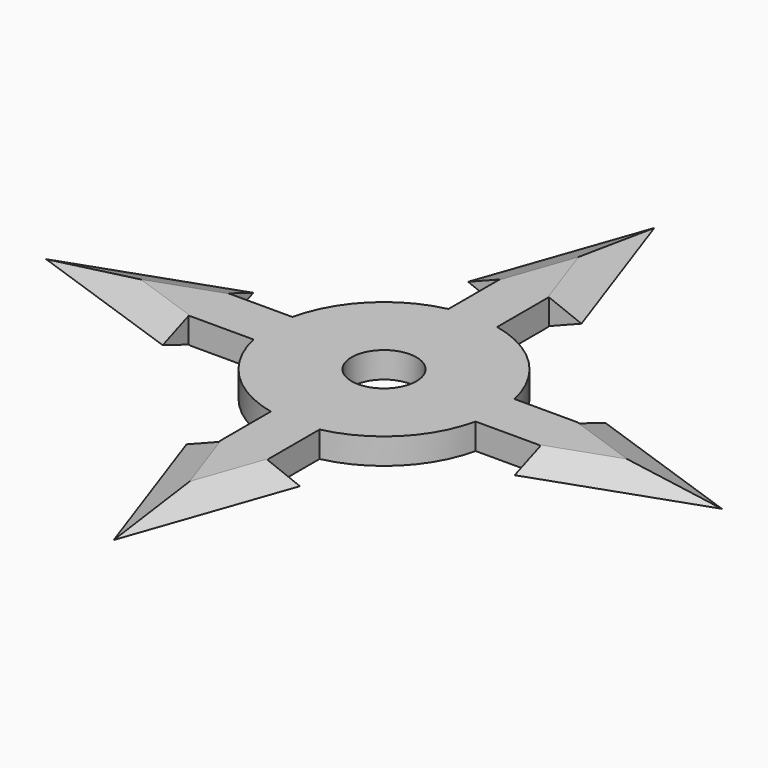
from build123d import *

# Parameters (mm, degrees)
F0_R         = 5
F1_DEPTH     = 2
F2_SIZE      = 1.99999
F3_T1_DEPTH  = 34.8509927222
F3_T3_DEPTH  = 34.8509927222
F3_T5_DEPTH  = 34.8509927222
F3_T7_DEPTH  = 34.8509927222
F3_T9_DEPTH  = 34.8509927222
F3_T11_DEPTH = 34.8509927222
F3_T13_DEPTH = 34.8509927222
F3_T15_DEPTH = 34.8509927222


# Not quite as in the source:
# - a fillet or chamfer that OpenCascade refuses, or shapes differently, is made with other operations: its cross-section is extruded or revolved along the edge and cut away or added
# - a fillet or chamfer is up to 0.001 mm smaller than in the source, because OpenCascade refuses the exact size


with BuildPart() as f1:
    # F0 (on Top) → F1 (new body, symmetric)
    with BuildSketch(Plane.XY):
        with BuildLine():
            ThreePointArc((17.093492914, -3.75), (17.3980764166, -1.8859843591), (17.5, 0))
            ThreePointArc((17.5, 0), (17.3980764166, 1.8859843591), (17.093492914, 3.75))
            ThreePointArc((17.093492914, 3.75), (12.3743686708, 12.3743686708), (3.75, 17.093492914))
            ThreePointArc((3.75, 17.093492914), (0, 17.5), (-3.75, 17.093492914))
            ThreePointArc((-3.75, 17.093492914), (-12.3743686708, 12.3743686708), (-17.093492914, 3.75))
            ThreePointArc((-17.093492914, 3.75), (-17.5, 0), (-17.093492914, -3.75))
            ThreePointArc((-17.093492914, -3.75), (-12.3743686708, -12.3743686708), (-3.75, -17.093492914))
            ThreePointArc((-3.75, -17.093492914), (0, -17.5), (3.75, -17.093492914))
            ThreePointArc((3.75, -17.093492914), (12.3743686708, -12.3743686708), (17.093492914, -3.75))
        make_face()
        Circle(F0_R, mode=Mode.SUBTRACT)
        with BuildLine():
            ThreePointArc((-17.093492914, -3.75), (-17.5, 0), (-17.093492914, 3.75))
            Line((-17.093492914, 3.75), (-27.093492914, 3.75))
            Line((-27.093492914, 3.75), (-27.093492914, -3.75))
            Line((-27.093492914, -3.75), (-17.093492914, -3.75))
        make_face()
        Polygon((-27.093492914, -3.75), (-27.093492914, 3.75), (-27.093492914, 8.75), (-52.093492914, 0), (-27.093492914, -8.75), align=None)
        with BuildLine():
            ThreePointArc((-3.75, 17.093492914), (0, 17.5), (3.75, 17.093492914))
            Line((3.75, 17.093492914), (3.75, 27.093492914))
            Line((3.75, 27.093492914), (-3.75, 27.093492914))
            Line((-3.75, 27.093492914), (-3.75, 17.093492914))
        make_face()
        Polygon((-3.75, 27.093492914), (3.75, 27.093492914), (8.75, 27.093492914), (0, 52.093492914), (-8.75, 27.093492914), align=None)
        Polygon((27.093492914, 8.75), (27.093492914, 3.75), (27.093492914, -3.75), (27.093492914, -8.75), (52.093492914, 0), align=None)
        Polygon((8.75, -27.093492914), (3.75, -27.093492914), (-3.75, -27.093492914), (-8.75, -27.093492914), (0, -52.093492914), align=None)
        with BuildLine():
            Line((3.75, -27.093492914), (3.75, -17.093492914))
            ThreePointArc((3.75, -17.093492914), (0, -17.5), (-3.75, -17.093492914))
            Line((-3.75, -17.093492914), (-3.75, -27.093492914))
            Line((-3.75, -27.093492914), (3.75, -27.093492914))
        make_face()
        with BuildLine():
            ThreePointArc((17.093492914, 3.75), (17.3980764166, 1.8859843591), (17.5, 0))
            ThreePointArc((17.5, 0), (17.3980764166, -1.8859843591), (17.093492914, -3.75))
            Line((17.093492914, -3.75), (27.093492914, -3.75))
            Line((27.093492914, -3.75), (27.093492914, 3.75))
            Line((27.093492914, 3.75), (17.093492914, 3.75))
        make_face()
    extrude(amount=F1_DEPTH, both=True)

    # F2 (size 2 in the source; OpenCascade refuses exactly that, so slightly less here)
    f2_edges = [f1.edges().sort_by_distance(p)[0] for p in [
        (4.375, -39.593493, 2),
        (-4.375, -39.593493, 2),
        (4.375, -39.593493, -2),
        (-4.375, -39.593493, -2),
        (39.593493, -4.375, -2),
        (39.593493, -4.375, 2),
        (39.593493, 4.375, 2),
        (-39.593493, -4.375, 2),
        (-39.593493, -4.375, -2),
        (-4.375, 39.593493, 2),
        (4.375, 39.593493, 2),
        (39.593493, 4.375, -2),
        (4.375, 39.593493, -2),
        (-39.593493, 4.375, 2),
        (-39.593493, 4.375, -2),
        (-4.375, 39.593493, -2),
    ]]
    chamfer(f2_edges, length=F2_SIZE)

    # F3: chamfer of 2.85 on 16 edges, made by hand

    # F3_s2 → F3_t1 (cut)
    with BuildSketch(Plane(origin=(-16.7962484861, -47.9892813888, 0), x_dir=(0, 0, 1), z_dir=(0.3303504247, 0.9438583564, 0))):
        Polygon((2, 12.3591175097), (-0.0152543264, 17.2243718361), (2, 15.2091175097), align=None)
        Polygon((-2, 12.3591175097), (0.0152543264, 17.2243718361), (-2, 15.2091175097), align=None)
    extrude(amount=F3_T1_DEPTH, mode=Mode.SUBTRACT)

    # F3_s4 → F3_t3 (cut)
    with BuildSketch(Plane(origin=(5.2832082381, -15.0948806803, 0), x_dir=(0, 0, 1), z_dir=(0.3303504247, -0.9438583564, 0))):
        Polygon((2, 12.3591175097), (-0.0152543264, 17.2243718361), (2, 15.2091175097), align=None)
        Polygon((-2, 12.3591175097), (0.0152543264, 17.2243718361), (-2, 15.2091175097), align=None)
    extrude(amount=F3_T3_DEPTH, mode=Mode.SUBTRACT)

    # F3_s6 → F3_t5 (cut)
    with BuildSketch(Plane(origin=(15.0948806803, 5.2832082381, 0), x_dir=(0, 0, 1), z_dir=(0.9438583564, 0.3303504247, 0))):
        Polygon((2, 12.3591175097), (-0.0152543264, 17.2243718361), (2, 15.2091175097), align=None)
        Polygon((-2, 12.3591175097), (0.0152543264, 17.2243718361), (-2, 15.2091175097), align=None)
    extrude(amount=F3_T5_DEPTH, mode=Mode.SUBTRACT)

    # F3_s8 → F3_t7 (cut)
    with BuildSketch(Plane(origin=(47.9892813888, -16.7962484861, 0), x_dir=(0, 0, 1), z_dir=(-0.9438583564, 0.3303504247, 0))):
        Polygon((2, 12.3591175097), (-0.0152543264, 17.2243718361), (2, 15.2091175097), align=None)
        Polygon((-2, 12.3591175097), (0.0152543264, 17.2243718361), (-2, 15.2091175097), align=None)
    extrude(amount=F3_T7_DEPTH, mode=Mode.SUBTRACT)

    # F3_s10 → F3_t9 (cut)
    with BuildSketch(Plane(origin=(-5.2832082381, 15.0948806803, 0), x_dir=(0, 0, 1), z_dir=(-0.3303504247, 0.9438583564, 0))):
        Polygon((2, 12.3591175097), (-0.0152543264, 17.2243718361), (2, 15.2091175097), align=None)
        Polygon((-2, 12.3591175097), (0.0152543264, 17.2243718361), (-2, 15.2091175097), align=None)
    extrude(amount=F3_T9_DEPTH, mode=Mode.SUBTRACT)

    # F3_s12 → F3_t11 (cut)
    with BuildSketch(Plane(origin=(16.7962484861, 47.9892813888, 0), x_dir=(0, 0, 1), z_dir=(-0.3303504247, -0.9438583564, 0))):
        Polygon((-0.0152543264, 17.2243718361), (2, 12.3591175097), (2, 15.2091175097), align=None)
        Polygon((0.0152543264, 17.2243718361), (-2, 12.3591175097), (-2, 15.2091175097), align=None)
    extrude(amount=F3_T11_DEPTH, mode=Mode.SUBTRACT)

    # F3_s14 → F3_t13 (cut)
    with BuildSketch(Plane(origin=(-15.0948806803, -5.2832082381, 0), x_dir=(0, 0, 1), z_dir=(-0.9438583564, -0.3303504247, 0))):
        Polygon((2, 12.3591175097), (-0.0152543264, 17.2243718361), (2, 15.2091175097), align=None)
        Polygon((-2, 12.3591175097), (0.0152543264, 17.2243718361), (-2, 15.2091175097), align=None)
    extrude(amount=F3_T13_DEPTH, mode=Mode.SUBTRACT)

    # F3_s16 → F3_t15 (cut)
    with BuildSketch(Plane(origin=(-47.9892813888, 16.7962484861, 0), x_dir=(0, 0, 1), z_dir=(0.9438583564, -0.3303504247, 0))):
        Polygon((2, 12.3591175097), (-0.0152543264, 17.2243718361), (2, 15.2091175097), align=None)
        Polygon((-2, 12.3591175097), (0.0152543264, 17.2243718361), (-2, 15.2091175097), align=None)
    extrude(amount=F3_T15_DEPTH, mode=Mode.SUBTRACT)


solid = f1.part
